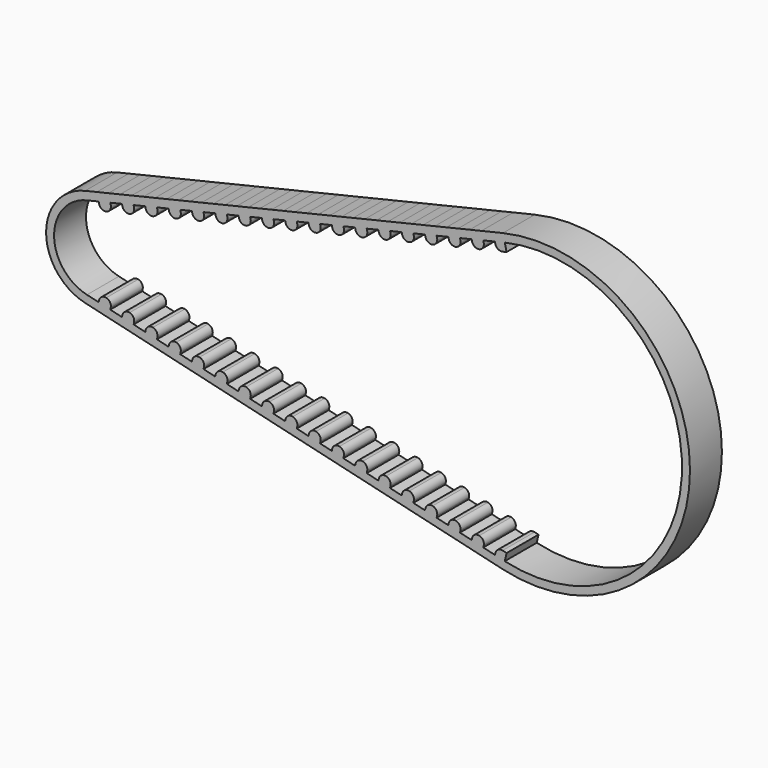
from build123d import *

# Parameters (mm, degrees)
F1_DEPTH = 10
F2_T     = -2
F3_W     = 3
F3_H     = 10
F3_W_2   = 2.5308332526
F4_DEPTH = 4
F5_R     = 1.5
F6_R     = 1.49999
F7_W     = 3
F7_H     = 10
F7_W_2   = 2.5308332526
F8_DEPTH = 4
F9_R     = 1.49999


# Not quite as in the source:
# - a fillet or chamfer is up to 0.001 mm smaller than in the source, because OpenCascade refuses the exact size


with BuildPart() as f1:
    # F0 (on Front) → F1 (new body)
    with BuildSketch(Plane.XZ):
        with BuildLine():
            Line((25.932428221, 37.0795976733), (-78.7184913193, 12.3598658911))
            ThreePointArc((-78.7184913193, 12.3598658911), (-88.4989510894, 0), (-78.7184913193, -12.3598658911))
            Line((-78.7184913193, -12.3598658911), (25.932428221, -37.0795976733))
            ThreePointArc((25.932428221, -37.0795976733), (72.7910489106, 0), (25.932428221, 37.0795976733))
        make_face()
    extrude(amount=F1_DEPTH)

    # F2
    f2_openings = [f1.faces().sort_by_distance(p)[0] for p in [
        (3.581658, -10, 0),
        (3.581658, 0, 0),
    ]]
    offset(amount=F2_T, openings=f2_openings)

    # F3 (on face) → F4 (join)
    with BuildSketch(Plane(origin=(-6.9252979833, 0, 29.3182308137), x_dir=(0.9732177867, 0, 0.2298850575), z_dir=(-0.2298850575, 0, 0.9732177867))):
        with Locations((-69.2688874135, -5)):
            Rectangle(F3_W, F3_H)
        with Locations((-63.2688874135, -5)):
            Rectangle(F3_W, F3_H)
        with Locations((-57.2688874135, -5)):
            Rectangle(F3_W, F3_H)
        with Locations((-51.2688874135, -5)):
            Rectangle(F3_W, F3_H)
        with Locations((-45.2688874135, -5)):
            Rectangle(F3_W, F3_H)
        with Locations((-39.2688874135, -5)):
            Rectangle(F3_W, F3_H)
        with Locations((-33.2688874135, -5)):
            Rectangle(F3_W, F3_H)
        with Locations((-27.2688874135, -5)):
            Rectangle(F3_W, F3_H)
        with Locations((-21.2688874135, -5)):
            Rectangle(F3_W, F3_H)
        with Locations((-15.2688874135, -5)):
            Rectangle(F3_W, F3_H)
        with Locations((-9.2688874135, -5)):
            Rectangle(F3_W, F3_H)
        with Locations((-3.2688874135, -5)):
            Rectangle(F3_W, F3_H)
        with Locations((2.7311125865, -5)):
            Rectangle(F3_W, F3_H)
        with Locations((8.7311125865, -5)):
            Rectangle(F3_W, F3_H)
        with Locations((14.7311125865, -5)):
            Rectangle(F3_W, F3_H)
        with Locations((20.7311125865, -5)):
            Rectangle(F3_W, F3_H)
        with Locations((26.7311125865, -5)):
            Rectangle(F3_W, F3_H)
        with Locations((32.4965292128, -5)):
            Rectangle(F3_W_2, F3_H)
    extrude(amount=-F4_DEPTH)

    # F5
    f5_edges = [f1.edges().sort_by_distance(p)[0] for p in [
        (-74.879298, -5, 9.15665),
    ]]
    fillet(f5_edges, radius=F5_R)

    # F6 (radius 1.5 in the source; OpenCascade refuses exactly that, so slightly less here)
    f6_edges = [f1.edges().sort_by_distance(p)[0] for p in [
        (-71.959644, -5, 9.846305),
        (-69.039991, -5, 10.53596),
        (-66.120338, -5, 11.225615),
        (-63.200684, -5, 11.915271),
        (-60.281031, -5, 12.604926),
        (-57.361378, -5, 13.294581),
        (-54.441724, -5, 13.984236),
        (-51.522071, -5, 14.673891),
        (-48.602417, -5, 15.363546),
        (-45.682764, -5, 16.053202),
        (-42.763111, -5, 16.742857),
        (-39.843457, -5, 17.432512),
        (-36.923804, -5, 18.122167),
        (-34.004151, -5, 18.811822),
        (-31.084497, -5, 19.501478),
        (-28.164844, -5, 20.191133),
        (-25.245191, -5, 20.880788),
        (-22.325537, -5, 21.570443),
        (-19.405884, -5, 22.260098),
        (-16.486231, -5, 22.949753),
        (-13.566577, -5, 23.639409),
        (-10.646924, -5, 24.329064),
        (-7.72727, -5, 25.018719),
        (-4.807617, -5, 25.708374),
        (-1.887964, -5, 26.398029),
        (1.03169, -5, 27.087684),
        (3.951343, -5, 27.77734),
        (6.870996, -5, 28.466995),
        (9.79065, -5, 29.15665),
        (12.710303, -5, 29.846305),
        (15.629956, -5, 30.53596),
        (18.54961, -5, 31.225615),
        (21.469263, -5, 31.915271),
        (24.388917, -5, 32.604926),
    ]]
    fillet(f6_edges, radius=F6_R)

    # F7 (on face) → F8 (join)
    with BuildSketch(Plane(origin=(-6.9252979833, 0, -29.3182308137), x_dir=(0.9732177867, 0, -0.2298850575), z_dir=(-0.2298850575, 0, -0.9732177867))):
        with Locations((-69.2688874135, 5)):
            Rectangle(F7_W, F7_H)
        with Locations((-63.2688874135, 5)):
            Rectangle(F7_W, F7_H)
        with Locations((-57.2688874135, 5)):
            Rectangle(F7_W, F7_H)
        with Locations((-51.2688874135, 5)):
            Rectangle(F7_W, F7_H)
        with Locations((-45.2688874135, 5)):
            Rectangle(F7_W, F7_H)
        with Locations((-39.2688874135, 5)):
            Rectangle(F7_W, F7_H)
        with Locations((-33.2688874135, 5)):
            Rectangle(F7_W, F7_H)
        with Locations((-27.2688874135, 5)):
            Rectangle(F7_W, F7_H)
        with Locations((-21.2688874135, 5)):
            Rectangle(F7_W, F7_H)
        with Locations((-15.2688874135, 5)):
            Rectangle(F7_W, F7_H)
        with Locations((-9.2688874135, 5)):
            Rectangle(F7_W, F7_H)
        with Locations((-3.2688874135, 5)):
            Rectangle(F7_W, F7_H)
        with Locations((2.7311125865, 5)):
            Rectangle(F7_W, F7_H)
        with Locations((8.7311125865, 5)):
            Rectangle(F7_W, F7_H)
        with Locations((14.7311125865, 5)):
            Rectangle(F7_W, F7_H)
        with Locations((20.7311125865, 5)):
            Rectangle(F7_W, F7_H)
        with Locations((26.7311125865, 5)):
            Rectangle(F7_W, F7_H)
        with Locations((32.4965292128, 5)):
            Rectangle(F7_W_2, F7_H)
    extrude(amount=-F8_DEPTH)

    # F9 (radius 1.5 in the source; OpenCascade refuses exactly that, so slightly less here)
    f9_edges = [f1.edges().sort_by_distance(p)[0] for p in [
        (-74.879298, -5, -9.15665),
        (-71.959644, -5, -9.846305),
        (-69.039991, -5, -10.53596),
        (-66.120338, -5, -11.225615),
        (-63.200684, -5, -11.915271),
        (-57.361378, -5, -13.294581),
        (-60.281031, -5, -12.604926),
        (-54.441724, -5, -13.984236),
        (-51.522071, -5, -14.673891),
        (-48.602417, -5, -15.363546),
        (-45.682764, -5, -16.053202),
        (-42.763111, -5, -16.742857),
        (-39.843457, -5, -17.432512),
        (-36.923804, -5, -18.122167),
        (-34.004151, -5, -18.811822),
        (-31.084497, -5, -19.501478),
        (-28.164844, -5, -20.191133),
        (-25.245191, -5, -20.880788),
        (-22.325537, -5, -21.570443),
        (-19.405884, -5, -22.260098),
        (-16.486231, -5, -22.949753),
        (-13.566577, -5, -23.639409),
        (-10.646924, -5, -24.329064),
        (-7.72727, -5, -25.018719),
        (-4.807617, -5, -25.708374),
        (-1.887964, -5, -26.398029),
        (1.03169, -5, -27.087684),
        (3.951343, -5, -27.77734),
        (6.870996, -5, -28.466995),
        (9.79065, -5, -29.15665),
        (12.710303, -5, -29.846305),
        (15.629956, -5, -30.53596),
        (18.54961, -5, -31.225615),
        (21.469263, -5, -31.915271),
        (24.388917, -5, -32.604926),
    ]]
    fillet(f9_edges, radius=F9_R)


solid = f1.part
